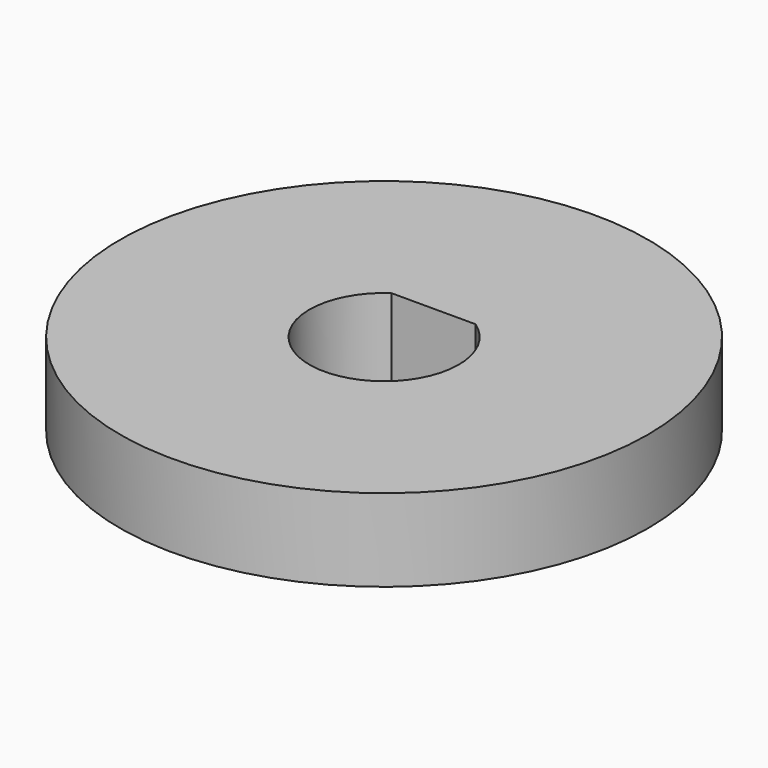
from build123d import *

# Parameters (mm, degrees)
F1_R     = 10.16
F2_DEPTH = 3.175


# Not quite as in the source:
# - a variable given as a bare number and used for a length is read in inches; the dataset says mm whatever the document's units were


with BuildPart() as f2:
    # F1 (on Top) → F2 (new body)
    with BuildSketch(Plane.XY):
        Circle(F1_R)
        with BuildLine():
            ThreePointArc((1.6195678436, 2.373), (0, -2.873), (-1.6195678436, 2.373))
            Line((-1.6195678436, 2.373), (0, 2.373))
            Line((0, 2.373), (1.6195678436, 2.373))
        make_face(mode=Mode.SUBTRACT)
    extrude(amount=F2_DEPTH)


solid = f2.part
